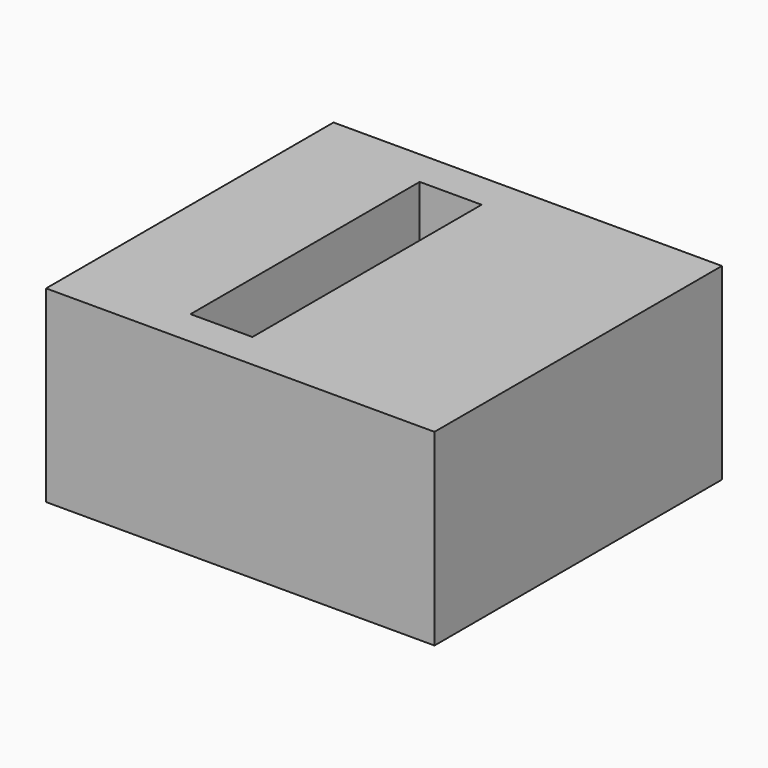
from build123d import *

# Parameters (mm, degrees)
F3_W     = 8.7
F3_H     = 11.8
F3_W_2   = 2.55
F3_W_3   = 4.75
F4_DEPTH = 3
F5_DEPTH = 7.75
F6_R     = 0.75
F7_DEPTH = 0.75
F8_R     = 0.7242640687
F9_DEPTH = 7.75


# Not quite as in the source:
# - a feature names something its author has since deleted; it is built from what else it names


with BuildPart() as f4:
    # F3 (on Top) → F4 (new body)
    with BuildSketch(Plane.XY):
        with Locations((3.65, 0)):
            Rectangle(F3_W, F3_H)
        with Locations((-1.975, 0)):
            Rectangle(F3_W_2, F3_H)
        with Locations((-5.625, 0)):
            Rectangle(F3_W_3, F3_H)
    extrude(amount=F4_DEPTH)

    # F3 (on Top) → F5 (join)
    with BuildSketch(Plane.XY):
        with Locations((3.65, 0)):
            Rectangle(F3_W, F3_H)
        Polygon((8, -7.4), (8, -5.9), (-0.7, -5.9), (-3.25, -5.9), (-8, -5.9), (-8, -7.4), align=None)
        Polygon((-0.7, 5.9), (8, 5.9), (8, 7.4), (-8, 7.4), (-8, 5.9), (-3.25, 5.9), align=None)
    extrude(amount=F5_DEPTH)

    # F6 (on face) → F7 (join)
    with BuildSketch(Plane(origin=(-0.7, 0, 0), x_dir=(0, -1, 0), z_dir=(-1, 0, 0))):
        with Locations((0, 5.75)):
            Circle(F6_R)
    extrude(amount=F7_DEPTH)

    # F8
    f8_edges = [f4.edges().sort_by_distance(p)[0] for p in [
        (-1.45, 0.75, 5.75),
    ]]
    fillet(f8_edges, radius=F8_R)

    # F3 (on Top) → F9 (join)
    with BuildSketch(Plane.XY):
        with Locations((-5.625, 0)):
            Rectangle(F3_W_3, F3_H)
    extrude(amount=F9_DEPTH)


solid = f4.part
